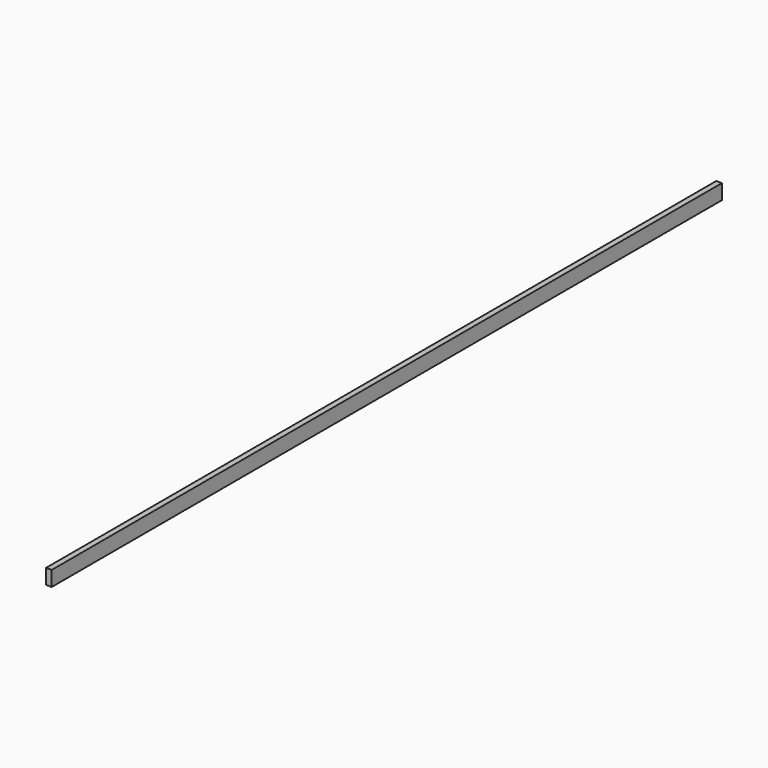
from build123d import *

# Parameters (mm, degrees)
F0_W     = 19.05
F0_H     = 50.8
F1_DEPTH = 2827.8666666667


# Not quite as in the source:
# - a length typed as a fraction of an inch, garbled in the dataset ("3 / 203.2 mm" for 3/8 in), is restored


with BuildPart() as f1:
    # F0 (on Front) → F1 (new body)
    with BuildSketch(Plane.XZ):
        with Locations((9.525, -25.4)):
            Rectangle(F0_W, F0_H)
    extrude(amount=F1_DEPTH)


solid = f1.part
